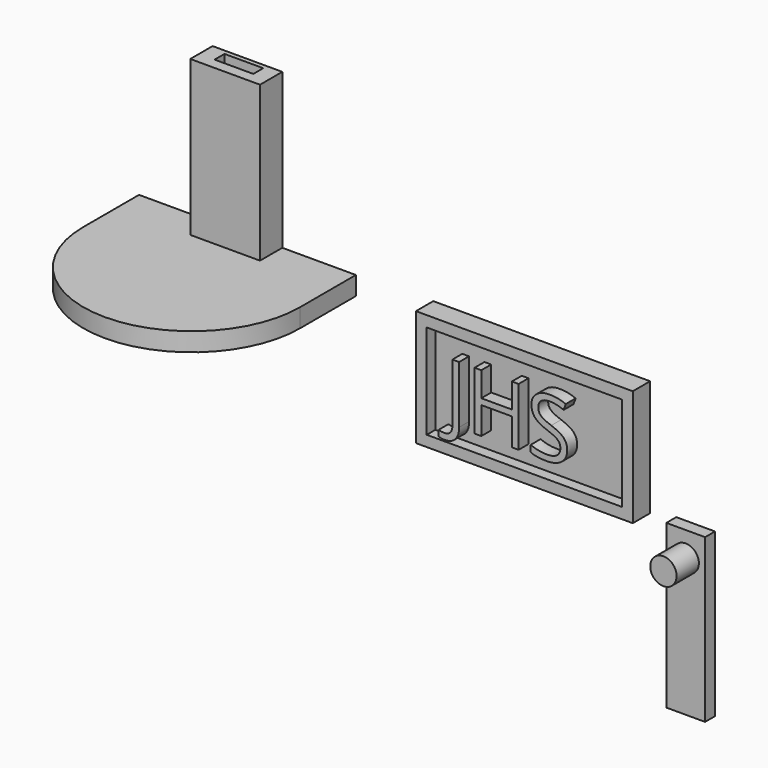
from build123d import *

# Parameters (mm, degrees)
F0_W         = 140
F0_H         = 75
F1_DEPTH     = 14
F2_T         = -7
F4_TEXT_SIZE = 52.4335903012
F5_DEPTH     = 8
F7_DEPTH     = 25
F8_R         = 8.5
F9_DEPTH     = 5
F10_W        = 25
F10_H        = 105
F11_DEPTH    = 8
F12_R        = 8.5
F13_DEPTH    = 18
F15_DEPTH    = 12
F17_DEPTH    = 100
F19_DEPTH    = 60


# Not quite as in the source:
# - Text() gives the source's letters only with a copy of the font that has no kerning and outlines rounded to 1/6400 em; it was checked with that copy


with BuildPart() as f1:
    # F0 (on Front) → F1 (new body)
    with BuildSketch(Plane.XZ):
        with Locations((-32.955661118, 5.8825448155)):
            Rectangle(F0_W, F0_H)
    extrude(amount=F1_DEPTH)

    # F2
    f2_openings = [f1.faces().sort_by_distance(p)[0] for p in [
        (-32.955661, -14, 5.882545),
    ]]
    offset(amount=F2_T, openings=f2_openings)

    # F4 (on offset) → F5 (join, through all)
    with BuildSketch(Plane.XZ.offset(15)):
        with Locations((-83.4492072463, -13.2295005023)):
            Text('JHS', F4_TEXT_SIZE, font='Open Sans', text_align=(TextAlign.LEFT, TextAlign.BOTTOM))
    extrude(amount=-F5_DEPTH)

    # F6 (on face) → F7 (join)
    with BuildSketch(Plane(origin=(0, 0, 0), x_dir=(-1, 0, 0), z_dir=(0, 1, 0))):
        Polygon((72.955661118, 23.0223227665), (32.955661118, 23.0223227665), (-7.044338882, 23.0223227665), (-7.044338882, -11.9776772335), (72.955661118, -11.9776772335), align=None)
    extrude(amount=F7_DEPTH)

    # F8 (on face) → F9 (cut)
    with BuildSketch(Plane(origin=(0, 25, 0), x_dir=(-1, 0, 0), z_dir=(0, 1, 0))):
        with Locations((32.955661118, 5.5223227665)):
            Circle(F8_R)
    extrude(amount=-F9_DEPTH, mode=Mode.SUBTRACT)


with BuildPart() as f11:
    # F10 (on Front) → F11 (new body)
    with BuildSketch(Plane.XZ):
        with Locations((66.4306387305, -80.8658695221)):
            Rectangle(F10_W, F10_H)
    extrude(amount=F11_DEPTH)

    # F12 (on face) → F13 (join)
    with BuildSketch(Plane.XZ.offset(8)):
        with Locations((66.4306387305, -44.4643907249)):
            Circle(F12_R)
    extrude(amount=F13_DEPTH)


with BuildPart() as f15:
    # F14 (on Top) → F15 (new body)
    with BuildSketch(Plane.XY):
        with BuildLine():
            Line((-188.8999199867, 45), (-328.8999199867, 45))
            Line((-328.8999199867, 45), (-328.8999199867, 0))
            ThreePointArc((-328.8999199867, 0), (-258.8999199867, -70), (-188.8999199867, 0))
            Line((-188.8999199867, 0), (-188.8999199867, 45))
        make_face()
    extrude(amount=F15_DEPTH)

    # F16 (on face) → F17 (join)
    with BuildSketch(Plane.XY.offset(12)):
        Polygon((-236.3999199867, 45), (-258.8999199867, 45), (-281.3999199867, 45), (-281.3999199867, 27), (-236.3999199867, 27), align=None)
    extrude(amount=F17_DEPTH)

    # F18 (on face) → F19 (cut)
    with BuildSketch(Plane.XY.offset(112)):
        Polygon((-246.3999199867, 42.0898782015), (-258.8999199867, 42.0898782015), (-271.3999199867, 42.0898782015), (-271.3999199867, 34.0898782015), (-246.3999199867, 34.0898782015), align=None)
    extrude(amount=-F19_DEPTH, mode=Mode.SUBTRACT)


solid = Compound([f1.part, f11.part, f15.part])
